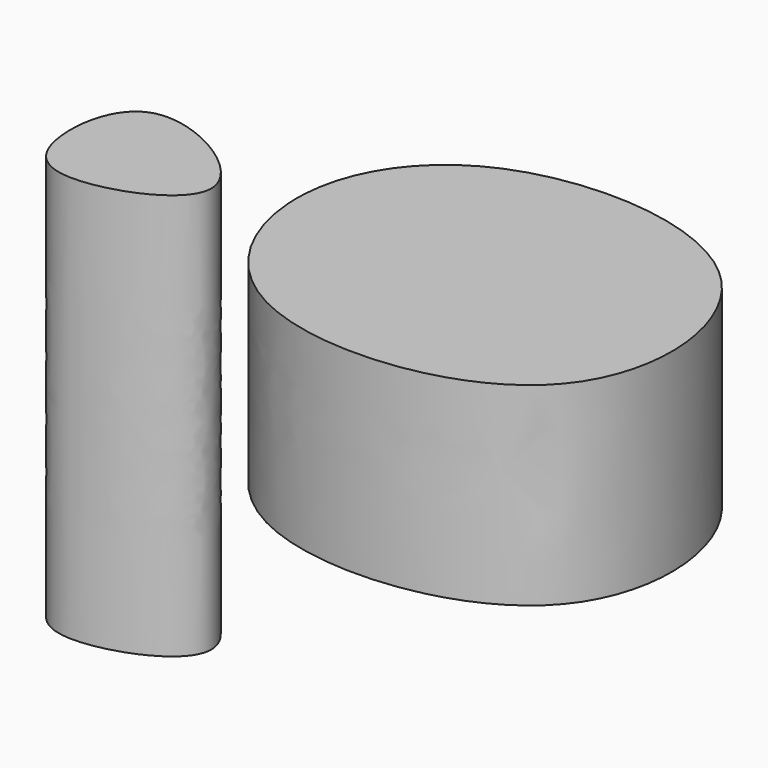
from build123d import *

# Parameters (mm, degrees)
F1_DEPTH = 22.098
F3_DEPTH = 46.228


with BuildPart() as f1:
    # F0 (on Top) → F1 (new body)
    with BuildSketch(Plane.XY):
        with BuildLine():
            add(Edge.make_bspline(
                [(-48.20728302, 24.9590966851), (-47.836216593, 31.3996072925), (-39.3940143743, 44.1088899766), (-3.8798088354, 41.4389580726), (-0.6624669754, 4.4911238271), (-40.8717736331, 0.8665344833), (-48.6067631615, 18.0254160776), (-48.20728302, 24.9590966851)],
                knots=[0, 0, 0, 0, 0.1735522435, 0.3894143581, 0.5907287191, 0.8131583196, 1, 1, 1, 1], degree=3))
        make_face()
    extrude(amount=F1_DEPTH)


with BuildPart() as f3:
    # F2 (on Top) → F3 (new body)
    with BuildSketch(Plane.XY):
        with BuildLine():
            add(Edge.make_bspline(
                [(-37.575765118, -21.75585535), (-40.771914841, -21.6333632841), (-44.3576469976, -17.8221725874), (-41.9547217235, -2.0678263136), (-18.6596234083, -16.2616017748), (-33.3237295059, -21.9188141197), (-37.575765118, -21.75585535)],
                knots=[0, 0, 0, 0, 0.2011470133, 0.4400462119, 0.7324016902, 1, 1, 1, 1], degree=3))
        make_face()
    extrude(amount=F3_DEPTH)


solid = Compound([f1.part, f3.part])
